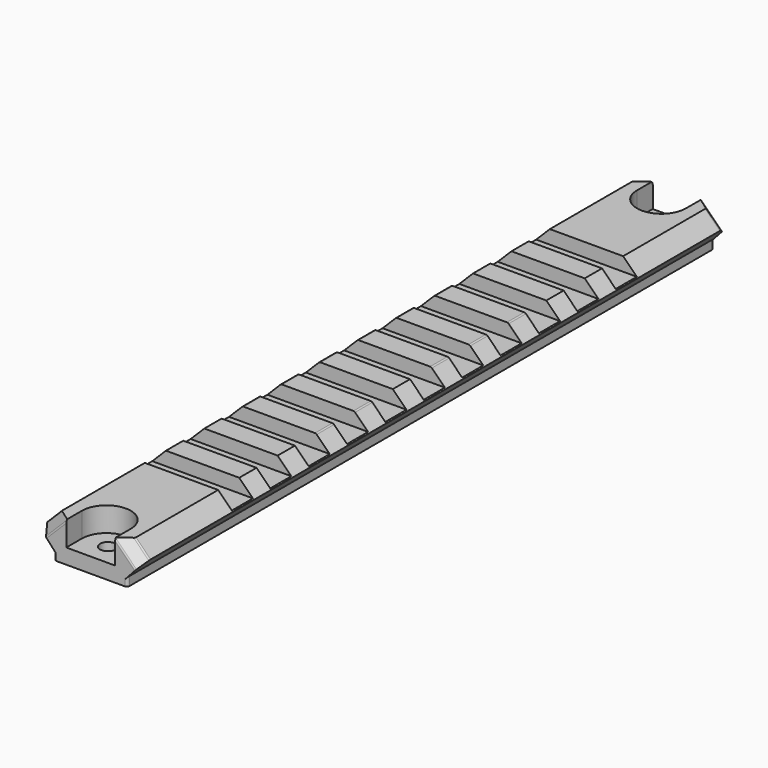
from build123d import *

# Parameters (mm, degrees)
F1_DEPTH = 75
F2_W     = 28
F2_H     = 5.4
F2_W_2   = 28.1193151165
F2_H_2   = 5.3996254659
F2_W_3   = 28.3288413435
F2_H_3   = 5.3951430639
F2_W_4   = 28.8207556829
F2_W_5   = 28.5256083831
F2_H_4   = 5.4125102987
F2_W_6   = 29.607820116
F2_W_7   = 29.9029674158
F3_DEPTH = 2.8
F5_DEPTH = 5
F6_R     = 1.6
F7_DEPTH = 3.101
F8_SIZE  = 2
F9_R     = 0.5


with BuildPart() as f1:
    # F0 (on Front) → F1 (new body, symmetric)
    with BuildSketch(Plane.XZ):
        Polygon((-7.5, -4.8), (7.5, -4.8), (7.5, -3), (10.5, 0.3), (7.5, 3.3), (-7.5, 3.3), (-10.5, 0.3), (-7.5, -3), align=None)
    extrude(amount=F1_DEPTH, both=True)

    # F2 (on face) → F3 (cut)
    with BuildSketch(Plane.XY.offset(3.3)):
        Rectangle(F2_W, F2_H)
        with Locations((0.0596575582, 9.8198127329)):
            Rectangle(F2_W_2, F2_H_2)
        with Locations((0.1644206718, 19.6375715319)):
            Rectangle(F2_W_3, F2_H_3)
        with Locations((0.4103778414, 29.46)):
            Rectangle(F2_W_4, F2_H)
        with Locations((0.2628041916, -9.8137448507)):
            Rectangle(F2_W_5, F2_H_4)
        with Locations((0.803910058, -19.6274897013)):
            Rectangle(F2_W_6, F2_H)
        with Locations((0.9514837079, -29.4474897013)):
            Rectangle(F2_W_7, F2_H)
        with Locations((0.4103778414, 39.28)):
            Rectangle(F2_W_4, F2_H)
        with Locations((0.4103778414, 49.1)):
            Rectangle(F2_W_4, F2_H)
        with Locations((0.9514837079, -39.2674897013)):
            Rectangle(F2_W_7, F2_H)
        with Locations((0.9514837079, -49.0874897013)):
            Rectangle(F2_W_7, F2_H)
    extrude(amount=-F3_DEPTH, mode=Mode.SUBTRACT)

    # F4 (on face) → F5 (cut)
    with BuildSketch(Plane.XY.offset(3.3)):
        with BuildLine():
            Line((-4.9999021515, -71), (-4.9999021515, -73))
            Line((-4.9999021515, -73), (-4.9999021515, -75))
            Line((-4.9999021515, -75), (5, -75))
            Line((5, -75), (5, -73))
            Line((5, -73), (5, -71))
            ThreePointArc((5, -71), (4.89242e-05, -66.0000489242), (-4.9999021515, -71))
        make_face()
        with BuildLine():
            ThreePointArc((-4.9999021515, 71), (4.89242e-05, 65.9778812301), (5, 71))
            Line((5, 71), (5, 73))
            Line((5, 73), (5, 75))
            Line((5, 75), (-4.9999021515, 75))
            Line((-4.9999021515, 75), (-4.9999021515, 73))
            Line((-4.9999021515, 73), (-4.9999021515, 71))
        make_face()
    extrude(amount=-F5_DEPTH, mode=Mode.SUBTRACT)

    # F6 (on face) → F7 (cut, through all)
    with BuildSketch(Plane.XY.offset(-1.7)):
        with Locations((0, -70.6000489272)):
            Circle(F6_R)
        with Locations((0, 70.5778812331)):
            Circle(F6_R)
    extrude(amount=-F7_DEPTH, mode=Mode.SUBTRACT)

    # F8
    f8_edges = [f1.edges().sort_by_distance(p)[0] for p in [
        (9, 75, 1.8),
        (-9, 75, 1.8),
        (9, -75, 1.8),
        (-9, -75, 1.8),
    ]]
    chamfer(f8_edges, length=F8_SIZE)

    # F9
    f9_edges = [f1.edges().sort_by_distance(p)[0] for p in [
        (-7.5, 24.547572, 3.3),
        (-7.5, 14.729813, 3.3),
        (-7.5, 4.91, 3.3),
        (-7.5, -4.903745, 3.3),
        (-7.5, -14.723745, 3.3),
        (-7.5, -24.53749, 3.3),
        (7.5, -24.53749, 3.3),
        (7.5, -14.723745, 3.3),
        (7.5, 4.91, 3.3),
        (7.5, 14.729813, 3.3),
        (7.5, 24.547572, 3.3),
        (-7.076516, 75, 0.895057),
        (9, 73, 1.8),
        (-9, 73, 1.8),
        (7.076565, -75, 0.895008),
        (9, -73, 1.8),
        (-7.076516, -75, 0.895057),
        (-9, -73, 1.8),
        (-7.5, -75, -3.9),
        (7.5, -75, -3.9),
        (7.5, 75, -3.9),
        (-7.5, 75, -3.9),
    ]]
    fillet(f9_edges, radius=F9_R)


solid = f1.part
